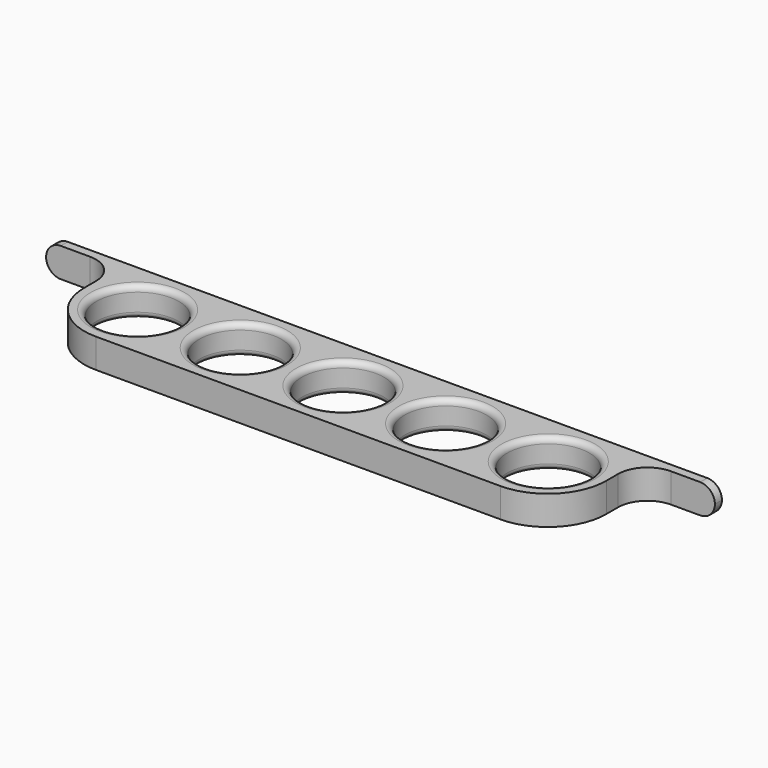
from build123d import *

# Parameters (mm, degrees)
F0_R     = 14
F1_DEPTH = 10
F2_R     = 2
F3_R     = 4.99999
F4_R     = 2


# Not quite as in the source:
# - a fillet or chamfer is up to 0.001 mm smaller than in the source, because OpenCascade refuses the exact size


with BuildPart() as f1:
    # F0 (on Top) → F1 (new body)
    with BuildSketch(Plane.XY):
        with BuildLine():
            Line((89, 19), (-89, 19))
            Line((-89, 19), (-114, 19))
            Line((-114, 19), (-114, 16))
            Line((-114, 16), (-99, 16))
            ThreePointArc((-99, 16), (-91.9289321881, 13.0710678119), (-89, 6))
            Line((-89, 6), (-89, 1))
            ThreePointArc((-89, 1), (-83.1421356237, -13.1421356237), (-69, -19))
            Line((-69, -19), (69, -19))
            ThreePointArc((69, -19), (83.1421356237, -13.1421356237), (89, 1))
            Line((89, 1), (89, 6))
            ThreePointArc((89, 6), (91.9289321881, 13.0710678119), (99, 16))
            Line((99, 16), (114, 16))
            Line((114, 16), (114, 19))
            Line((114, 19), (89, 19))
        make_face()
        with Locations((-70, 0)):
            Circle(F0_R, mode=Mode.SUBTRACT)
        with Locations((-35, 0)):
            Circle(F0_R, mode=Mode.SUBTRACT)
        Circle(F0_R, mode=Mode.SUBTRACT)
        with Locations((35, 0)):
            Circle(F0_R, mode=Mode.SUBTRACT)
        with Locations((70, 0)):
            Circle(F0_R, mode=Mode.SUBTRACT)
    extrude(amount=F1_DEPTH)

    # F2
    f2_edges = [f1.edges().sort_by_distance(p)[0] for p in [
        (-84, 0, 10),
        (-49, 0, 10),
        (-14, 0, 10),
        (21, 0, 10),
        (56, 0, 10),
    ]]
    fillet(f2_edges, radius=F2_R)

    # F3 (radius 5 in the source; OpenCascade refuses exactly that, so slightly less here)
    f3_edges = [f1.edges().sort_by_distance(p)[0] for p in [
        (-114, 17.5, 10),
        (-114, 17.5, 0),
        (114, 17.5, 10),
        (114, 17.5, 0),
    ]]
    fillet(f3_edges, radius=F3_R)

    # F4
    f4_edges = [f1.edges().sort_by_distance(p)[0] for p in [
        (56, 0, 0),
        (21, 0, 0),
        (-14, 0, 0),
        (-49, 0, 0),
        (-84, 0, 0),
    ]]
    fillet(f4_edges, radius=F4_R)


solid = f1.part
